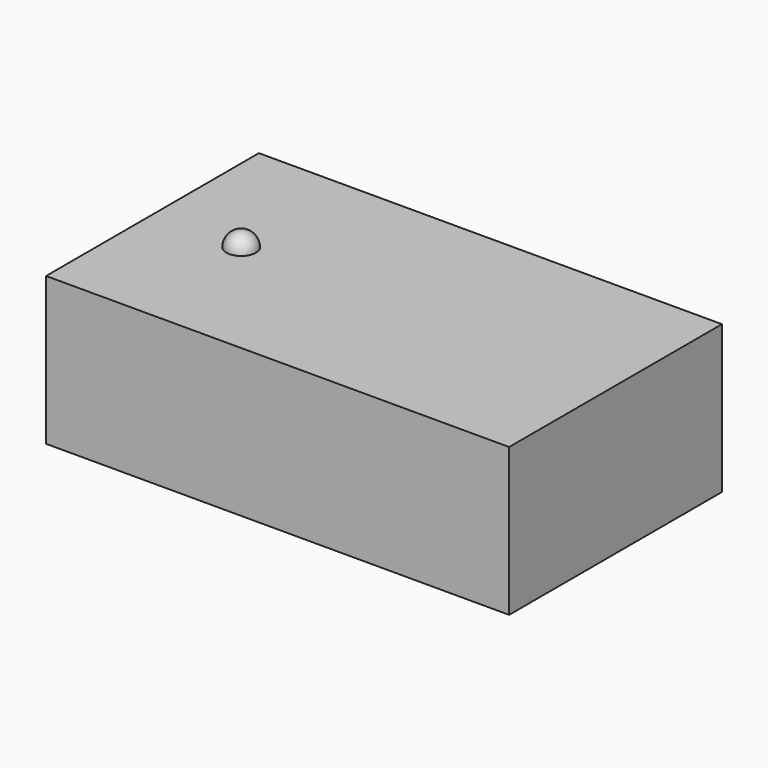
from build123d import *

# Parameters (mm, degrees)
F0_W     = 47
F0_H     = 15
F1_DEPTH = 27
F2_R     = 1.5
F3_DEPTH = 1.5
F4_R     = 1.49999


# Not quite as in the source:
# - a fillet or chamfer is up to 0.001 mm smaller than in the source, because OpenCascade refuses the exact size


with BuildPart() as f1:
    # F0 (on Front) → F1 (new body)
    with BuildSketch(Plane.XZ):
        with Locations((23.5, 7.5)):
            Rectangle(F0_W, F0_H)
    extrude(amount=F1_DEPTH)

    # F2 (on face) → F3 (join)
    with BuildSketch(Plane.XY.offset(15)):
        with Locations((9, -13.5)):
            Circle(F2_R)
    extrude(amount=F3_DEPTH)

    # F4 (radius 1.5 in the source; OpenCascade refuses exactly that, so slightly less here)
    f4_edges = [f1.edges().sort_by_distance(p)[0] for p in [
        (7.5, -13.5, 16.5),
    ]]
    fillet(f4_edges, radius=F4_R)


solid = f1.part
